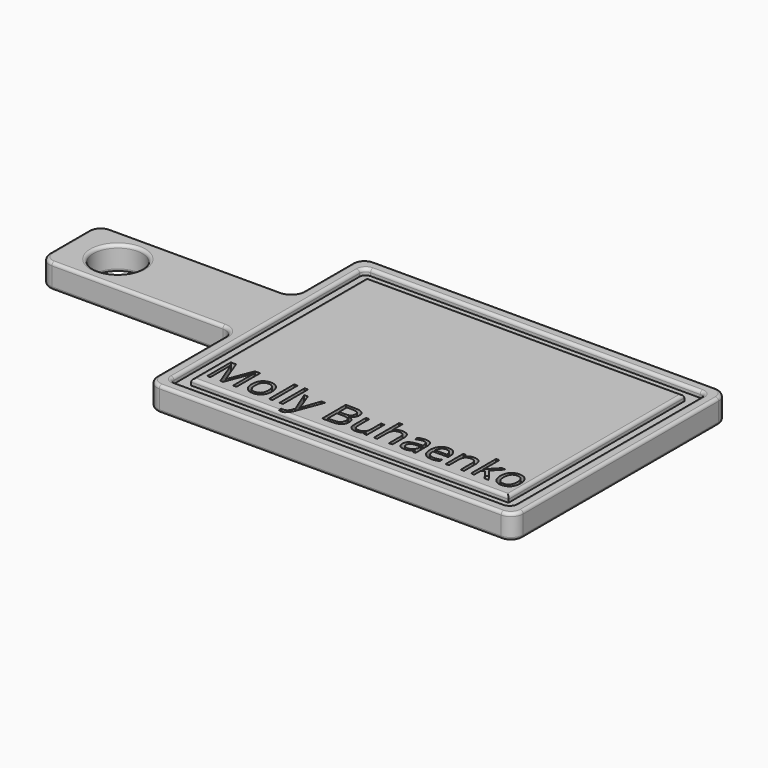
from build123d import *

# Parameters (mm, degrees)
F0_W         = 203.2
F0_H         = 76.2
F1_DEPTH     = 25.4
F2_R         = 25.4
F3_DEPTH     = 25.4
F5_DEPTH     = 6.35
F6_R         = 6.35
F7_R         = 12.7
F8_R         = 3.175
F9_TEXT_SIZE = 43.0624774835
F10_DEPTH    = 6.35


# Not quite as in the source:
# - Text() gives the source's letters only with a copy of the font that has no kerning and outlines rounded to 1/6400 em; it was checked with that copy


with BuildPart() as f1:
    # F0 (on Top) → F1 (new body)
    with BuildSketch(Plane.XY):
        Polygon((0, 114.3), (0, 0), (381, 0), (381, 279.4), (0, 279.4), (0, 190.5), align=None)
        with Locations((-101.6, 152.4)):
            Rectangle(F0_W, F0_H)
    extrude(amount=F1_DEPTH)

    # F2 (on face) → F3 (cut)
    with BuildSketch(Plane.XY.offset(25.4)):
        with Locations((-152.4, 152.4)):
            Circle(F2_R)
    extrude(amount=-F3_DEPTH, mode=Mode.SUBTRACT)

    # F4 (on face) → F5 (cut)
    with BuildSketch(Plane.XY.offset(25.4)):
        Polygon((12.7000004292, 114.3), (12.7000004292, 12.7000004292), (368.2999995708, 12.7000004292), (368.2999995708, 266.6999995708), (12.7000004292, 266.6999995708), (12.7000004292, 190.5), align=None)
        Polygon((25.3999918938, 114.3), (25.3999918938, 190.5), (25.3999918938, 254.0000081062), (355.6000081062, 254.0000081062), (355.6000081062, 25.3999918938), (25.3999918938, 25.3999918938), align=None, mode=Mode.SUBTRACT)
    extrude(amount=-F5_DEPTH, mode=Mode.SUBTRACT)

    # F6
    f6_edges = [f1.edges().sort_by_distance(p)[0] for p in [
        (12.7, 266.7, 22.225),
        (368.3, 12.7, 22.225),
        (12.7, 12.7, 22.225),
        (368.3, 266.7, 22.225),
    ]]
    fillet(f6_edges, radius=F6_R)

    # F7
    f7_edges = [f1.edges().sort_by_distance(p)[0] for p in [
        (-203.2, 114.3, 12.7),
        (-203.2, 190.5, 12.7),
        (0, 0, 12.7),
        (381, 0, 12.7),
        (381, 279.4, 12.7),
        (0, 279.4, 12.7),
        (0, 190.5, 12.7),
        (0, 114.3, 12.7),
    ]]
    fillet(f7_edges, radius=F7_R)

    # F8
    f8_edges = [f1.edges().sort_by_distance(p)[0] for p in [
        (190.5, 254.000008, 25.4),
        (355.600008, 139.7, 25.4),
        (190.5, 25.399992, 25.4),
        (25.399992, 139.7, 25.4),
        (0, 57.15, 0),
        (-3.719744, 110.580256, 0),
        (3.719744, 3.719744, 0),
        (-101.6, 114.3, 0),
        (190.5, 0, 0),
        (-199.480256, 118.019744, 0),
        (377.280256, 3.719744, 0),
        (-203.2, 152.4, 0),
        (381, 139.7, 0),
        (-199.480256, 186.780256, 0),
        (377.280256, 275.680256, 0),
        (-101.6, 190.5, 0),
        (190.5, 279.4, 0),
        (-3.719744, 194.219744, 0),
        (3.719744, 275.680256, 0),
        (0, 234.95, 0),
        (-177.8, 152.4, 0),
        (0, 57.15, 25.4),
        (-3.719744, 110.580256, 25.4),
        (3.719744, 3.719744, 25.4),
        (-101.6, 114.3, 25.4),
        (190.5, 0, 25.4),
        (-199.480256, 118.019744, 25.4),
        (377.280256, 3.719744, 25.4),
        (-203.2, 152.4, 25.4),
        (381, 139.7, 25.4),
        (-199.480256, 186.780256, 25.4),
        (377.280256, 275.680256, 25.4),
        (-101.6, 190.5, 25.4),
        (190.5, 279.4, 25.4),
        (-3.719744, 194.219744, 25.4),
        (3.719744, 275.680256, 25.4),
        (0, 234.95, 25.4),
        (190.5, 12.7, 25.4),
        (14.559872, 14.559872, 25.4),
        (366.440128, 14.559872, 25.4),
        (12.7, 139.7, 25.4),
        (368.3, 139.7, 25.4),
        (14.559872, 264.840128, 25.4),
        (366.440128, 264.840128, 25.4),
        (190.5, 266.7, 25.4),
        (-177.8, 152.4, 25.4),
    ]]
    fillet(f8_edges, radius=F8_R)

    # F9 (on face) → F10 (cut)
    with BuildSketch(Plane.XY.offset(25.4)):
        with Locations((28.5749918938, 37.0994521163)):
            Text('Molly Buhaenko', F9_TEXT_SIZE, font='Open Sans', text_align=(TextAlign.LEFT, TextAlign.BOTTOM))
    extrude(amount=-F10_DEPTH, mode=Mode.SUBTRACT)


solid = f1.part
